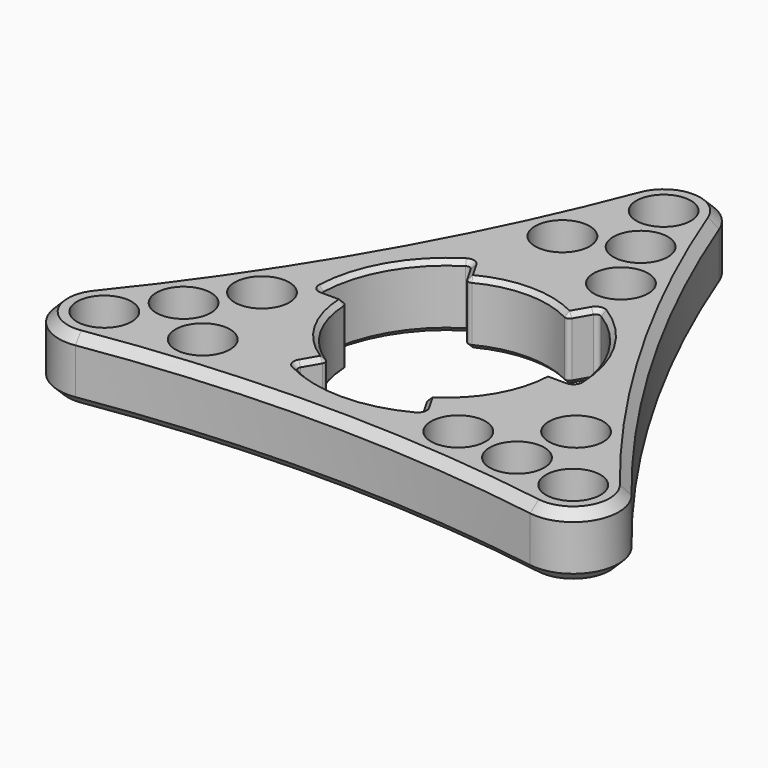
from build123d import *

# Parameters (mm, degrees)
F0_R     = 3
F1_DEPTH = 7
F2_R     = 5
F3_R     = 0.5
F4_SIZE  = 0.49999
F5_DEPTH = 2
F6_SIZE  = 1
F7_R     = 1
F8_DEPTH = 25


# Not quite as in the source:
# - a fillet or chamfer is up to 0.001 mm smaller than in the source, because OpenCascade refuses the exact size
# - a feature names something its author has since deleted; it is built from what else it names


with BuildPart() as f1:
    # F0 (on Top) → F1 (new body)
    with BuildSketch(Plane.XY):
        with BuildLine():
            ThreePointArc((39.4776041315, -22.7924053723), (15.4655621526, 8.929046472), (0, 45.5848107446))
            ThreePointArc((0, 45.5848107446), (-15.4655621526, 8.929046472), (-39.4776041315, -22.7924053723))
            ThreePointArc((-39.4776041315, -22.7924053723), (0, -17.858092944), (39.4776041315, -22.7924053723))
        make_face()
        with Locations((-25.7694508258, -14.8779993712)):
            Circle(F0_R, mode=Mode.SUBTRACT)
        with Locations((-21.4838139861, -9.3432620804)):
            Circle(F0_R, mode=Mode.SUBTRACT)
        with Locations((-15.9490766953, -13.6288989201)):
            Circle(F0_R, mode=Mode.SUBTRACT)
        with Locations((-17.4362165574, -3.6321365298)):
            Circle(F0_R, mode=Mode.SUBTRACT)
        with Locations((11.8636307835, -13.2841382197)):
            Circle(F0_R, mode=Mode.SUBTRACT)
        with Locations((18.8334093089, -13.933897642)):
            Circle(F0_R, mode=Mode.SUBTRACT)
        with Locations((25.7694508258, -14.8779993712)):
            Circle(F0_R, mode=Mode.SUBTRACT)
        with Locations((19.7775110381, -6.997856125)):
            Circle(F0_R, mode=Mode.SUBTRACT)
        with BuildLine():
            ThreePointArc((7, 12.124355653), (12.124355653, 7), (14, 0))
            ThreePointArc((14, 0), (12.124355653, -7), (7, -12.124355653))
            ThreePointArc((7, -12.124355653), (0, -14), (-7, -12.124355653))
            ThreePointArc((-7, -12.124355653), (-12.124355653, -7), (-14, 0))
            ThreePointArc((-14, 0), (-12.124355653, 7), (-7, 12.124355653))
            ThreePointArc((-7, 12.124355653), (0, 14), (7, 12.124355653))
        make_face(mode=Mode.SUBTRACT)
        with Locations((-3.8284343428, 20.6267550451)):
            Circle(F0_R, mode=Mode.SUBTRACT)
        with Locations((5.5725857739, 16.9162747495)):
            Circle(F0_R, mode=Mode.SUBTRACT)
        with Locations((2.6504046772, 23.2771597223)):
            Circle(F0_R, mode=Mode.SUBTRACT)
        with Locations((0, 29.7559987423)):
            Circle(F0_R, mode=Mode.SUBTRACT)
        with BuildLine():
            ThreePointArc((-5.5, 9.5262794416), (0, 11), (5.5, 9.5262794416))
            Line((5.5, 9.5262794416), (7, 12.124355653))
            ThreePointArc((7, 12.124355653), (0, 14), (-7, 12.124355653))
            Line((-7, 12.124355653), (-5.5, 9.5262794416))
        make_face()
        with BuildLine():
            Line((-7, -12.124355653), (-5.5, -9.5262794416))
            ThreePointArc((-5.5, -9.5262794416), (-9.5262794416, -5.5), (-11, 0))
            Line((-11, 0), (-14, 0))
            ThreePointArc((-14, 0), (-12.124355653, -7), (-7, -12.124355653))
        make_face()
        with BuildLine():
            Line((14, 0), (11, 0))
            ThreePointArc((11, 0), (9.5262794416, -5.5), (5.5, -9.5262794416))
            Line((5.5, -9.5262794416), (7, -12.124355653))
            ThreePointArc((7, -12.124355653), (12.124355653, -7), (14, 0))
        make_face()
    extrude(amount=F1_DEPTH)

    # F2
    f2_edges = [f1.edges().sort_by_distance(p)[0] for p in [
        (39.477604, -22.792405, 3.5),
        (-39.477604, -22.792405, 3.5),
        (0, 45.584811, 3.5),
    ]]
    fillet(f2_edges, radius=F2_R)

    # F3
    f3_edges = [f1.edges().sort_by_distance(p)[0] for p in [
        (-7, 12.124356, 3.5),
        (-5.5, 9.526279, 3.5),
        (5.5, 9.526279, 3.5),
        (7, 12.124356, 3.5),
        (14, 0, 3.5),
        (11, 0, 3.5),
        (5.5, -9.526279, 3.5),
        (7, -12.124356, 3.5),
        (-14, 0, 3.5),
        (-11, 0, 3.5),
        (-7, -12.124356, 3.5),
        (-5.5, -9.526279, 3.5),
    ]]
    fillet(f3_edges, radius=F3_R)

    # F4 (size 0.5 in the source; OpenCascade refuses exactly that, so slightly less here)
    f4_edges = [f1.edges().sort_by_distance(p)[0] for p in [
        (9.526279, -5.5, 0),
        (9.526279, -5.5, 7),
    ]]
    chamfer(f4_edges, length=F4_SIZE)

    # F0 (on Top) → F5 (join)
    with BuildSketch(Plane.XY):
        with Locations((0, 29.7559987423)):
            Circle(F0_R)
        with Locations((2.6504046772, 23.2771597223)):
            Circle(F0_R)
        with Locations((5.5725857739, 16.9162747495)):
            Circle(F0_R)
        with Locations((-3.8284343428, 20.6267550451)):
            Circle(F0_R)
        with Locations((-17.4362165574, -3.6321365298)):
            Circle(F0_R)
        with Locations((-21.4838139861, -9.3432620804)):
            Circle(F0_R)
        with Locations((-25.7694508258, -14.8779993712)):
            Circle(F0_R)
        with Locations((-15.9490766953, -13.6288989201)):
            Circle(F0_R)
        with Locations((11.8636307835, -13.2841382197)):
            Circle(F0_R)
        with Locations((18.8334093089, -13.933897642)):
            Circle(F0_R)
        with Locations((25.7694508258, -14.8779993712)):
            Circle(F0_R)
        with Locations((19.7775110381, -6.997856125)):
            Circle(F0_R)
    extrude(amount=F5_DEPTH)

    # F6
    f6_edges = [f1.edges().sort_by_distance(p)[0] for p in [
        (0, -17.858093, 0),
        (0, -17.858093, 7),
    ]]
    chamfer(f6_edges, length=F6_SIZE)

    # F7
    f7_edges = [f1.edges().sort_by_distance(p)[0] for p in [
        (-28.769451, -14.877999, 2),
        (-24.483814, -9.343262, 2),
        (-20.436217, -3.632137, 2),
        (-18.949077, -13.628899, 2),
        (-6.828434, 20.626755, 2),
        (-3, 29.755999, 2),
        (-0.349595, 23.27716, 2),
        (2.572586, 16.916275, 2),
        (16.777511, -6.997856, 2),
        (8.863631, -13.284138, 2),
        (15.833409, -13.933898, 2),
        (22.769451, -14.877999, 2),
    ]]
    fillet(f7_edges, radius=F7_R)

    # F8 (cut): faces of the model
    f8_faces = [f1.faces().sort_by_distance(p)[0] for p in [
        (25.7694508258, -14.8779993712, 2),
        (18.8334093089, -13.933897642, 2),
        (19.7775110381, -6.997856125, 2),
        (11.8636307835, -13.2841382197, 2),
        (5.5725857739, 16.9162747495, 2),
        (2.6504046772, 23.2771597223, 2),
        (0, 29.7559987423, 2),
        (-3.8284343428, 20.6267550451, 2),
        (-17.4362165574, -3.6321365298, 2),
        (-21.4838139861, -9.3432620804, 2),
        (-25.7694508258, -14.8779993712, 2),
        (-15.9490766953, -13.6288989201, 2),
    ]]
    extrude(f8_faces, amount=-F8_DEPTH, mode=Mode.SUBTRACT)


solid = f1.part
